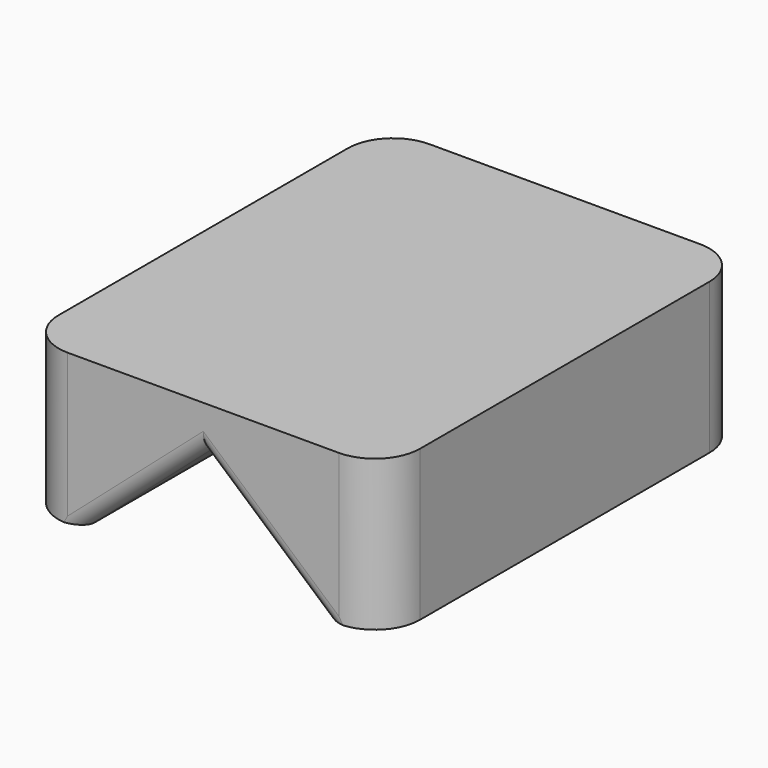
from build123d import *

# Parameters (mm, degrees)
F1_DEPTH     = 15
F2_R         = 1.5
F3_T4_DEPTH  = 7.8150729064
F3_T9_DEPTH  = 7.8150729064
F3_T14_DEPTH = 7.8150729064
F3_T19_DEPTH = 7.8150729064
F3_T25_DEPTH = 7.8150729064
F3_T29_DEPTH = 7.8150729064
F3_T36_DEPTH = 7.8150729064
F3_T40_DEPTH = 7.8150729064


# Not quite as in the source:
# - a fillet or chamfer that OpenCascade refuses, or shapes differently, is made with other operations: its cross-section is extruded or revolved along the edge and cut away or added


with BuildPart() as f1:
    # F0 (on Front) → F1 (new body)
    with BuildSketch(Plane.XZ):
        Polygon((0, 5), (0, 0), (2, 0), (6, 3.5), (10, 0), (12, 0), (12, 5), align=None)
    extrude(amount=F1_DEPTH)

    # F2
    f2_edges = [f1.edges().sort_by_distance(p)[0] for p in [
        (0, -15, 2.5),
        (12, -15, 2.5),
        (12, 0, 2.5),
        (0, 0, 2.5),
    ]]
    fillet(f2_edges, radius=F2_R)

    # F3: fillet of radius 0.5 on 4 edges, made by hand


with BuildPart() as f3_tool2:
    # F3_s3 → F3_t4 (new body)
    with BuildSketch(Plane(origin=(0.1920224944, 0, 0.1680196826), x_dir=(0, 1, 0), z_dir=(0.7525766947, 0, 0.6585046079))):
        with BuildLine():
            ThreePointArc((-15, -0.8170092157), (-14.8535533906, -1.1705626063), (-14.5, -1.3170092157))
            Line((-14.5, -1.3170092157), (-15, -1.3170092157))
            Line((-15, -1.3170092157), (-15, -0.8170092157))
        make_face()
    extrude(amount=F3_T4_DEPTH)

    split(bisect_by=Plane(origin=(4.3362831858, 0, 4.9557522124), x_dir=(0, 1, 0), z_dir=(-0.6585046079, 0, -0.7525766947)), keep=Keep.TOP)


with BuildPart() as f1_1:
    add(f1.part)

    # F3_t1: cut F3_tool2
    add(f3_tool2.part, mode=Mode.SUBTRACT)


with BuildPart() as f3_tool7:
    # F3_s8 → F3_t9 (new body)
    with BuildSketch(Plane(origin=(0.7229959458, 0, -0.6326214526), x_dir=(0, 1, 0), z_dir=(0.7525766947, 0, -0.6585046079))):
        with BuildLine():
            ThreePointArc((-15, 7.0850460787), (-14.8535533906, 6.7314926881), (-14.5, 6.5850460787))
            Line((-14.5, 6.5850460787), (-15, 6.5850460787))
            Line((-15, 6.5850460787), (-15, 7.0850460787))
        make_face()
    extrude(amount=F3_T9_DEPTH)

    split(bisect_by=Plane(origin=(0.8672566372, 0, -0.9911504425), x_dir=(0, 1, 0), z_dir=(0.6585046079, 0, -0.7525766947)), keep=Keep.TOP)


with BuildPart() as f1_2:
    add(f1_1.part)

    # F3_t6: cut F3_tool7
    add(f3_tool7.part, mode=Mode.SUBTRACT)


with BuildPart() as f3_tool12:
    # F3_s13 → F3_t14 (new body)
    with BuildSketch(Plane(origin=(0.1920224944, 0, 0.1680196826), x_dir=(0, 1, 0), z_dir=(0.7525766947, 0, 0.6585046079))):
        with BuildLine():
            ThreePointArc((0, -0.8170092157), (-0.1464466094, -1.1705626063), (-0.5, -1.3170092157))
            Line((-0.5, -1.3170092157), (0, -1.3170092157))
            Line((0, -1.3170092157), (0, -0.8170092157))
        make_face()
    extrude(amount=F3_T14_DEPTH)

    split(bisect_by=Plane(origin=(4.3362831858, 0, 4.9557522124), x_dir=(0, 1, 0), z_dir=(-0.6585046079, 0, -0.7525766947)), keep=Keep.TOP)


with BuildPart() as f1_3:
    add(f1_2.part)

    # F3_t11: cut F3_tool12
    add(f3_tool12.part, mode=Mode.SUBTRACT)


with BuildPart() as f3_tool17:
    # F3_s18 → F3_t19 (new body)
    with BuildSketch(Plane(origin=(0.7229959458, 0, -0.6326214526), x_dir=(0, 1, 0), z_dir=(0.7525766947, 0, -0.6585046079))):
        with BuildLine():
            ThreePointArc((0, 7.0850460787), (-0.1464466094, 6.7314926881), (-0.5, 6.5850460787))
            Line((-0.5, 6.5850460787), (0, 6.5850460787))
            Line((0, 6.5850460787), (0, 7.0850460787))
        make_face()
    extrude(amount=F3_T19_DEPTH)

    split(bisect_by=Plane(origin=(0.8672566372, 0, -0.9911504425), x_dir=(0, 1, 0), z_dir=(0.6585046079, 0, -0.7525766947)), keep=Keep.TOP)


with BuildPart() as f1_4:
    add(f1_3.part)

    # F3_t16: cut F3_tool17
    add(f3_tool17.part, mode=Mode.SUBTRACT)


with BuildPart() as f3_tool23:
    # F3_s24 → F3_t25 (new body)
    with BuildSketch(Plane(origin=(0.1920224944, 0, 0.1680196826), x_dir=(0, 1, 0), z_dir=(0.7525766947, 0, 0.6585046079))):
        with BuildLine():
            ThreePointArc((-15, -0.8170092157), (-14.8535533906, -1.1705626063), (-14.5, -1.3170092157))
            Line((-14.5, -1.3170092157), (-15, -1.3170092157))
            Line((-15, -1.3170092157), (-15, -0.8170092157))
        make_face()
    extrude(amount=F3_T25_DEPTH)

    split(bisect_by=Plane(origin=(4.3362831858, 0, 4.9557522124), x_dir=(0, 1, 0), z_dir=(0.6585046079, 0, 0.7525766947)), keep=Keep.TOP)


with BuildPart() as f3_tool27:
    # F3_s28 → F3_t29 (new body)
    with BuildSketch(Plane(origin=(0.7229959458, 0, -0.6326214526), x_dir=(0, 1, 0), z_dir=(0.7525766947, 0, -0.6585046079))):
        with BuildLine():
            ThreePointArc((-15, 7.0850460787), (-14.8535533906, 6.7314926881), (-14.5, 6.5850460787))
            Line((-14.5, 6.5850460787), (-15, 6.5850460787))
            Line((-15, 6.5850460787), (-15, 7.0850460787))
        make_face()
    extrude(amount=F3_T29_DEPTH)

    split(bisect_by=Plane(origin=(0.8672566372, 0, -0.9911504425), x_dir=(0, 1, 0), z_dir=(-0.6585046079, 0, 0.7525766947)), keep=Keep.TOP)


with BuildPart() as f3_tool23_1:
    add(f3_tool23.part)

    # F3_t31: intersect F3_tool27
    add(f3_tool27.part, mode=Mode.INTERSECT)


with BuildPart() as f1_5:
    add(f1_4.part)

    # F3_t21: cut F3_tool23
    add(f3_tool23_1.part, mode=Mode.SUBTRACT)


with BuildPart() as f3_tool34:
    # F3_s35 → F3_t36 (new body)
    with BuildSketch(Plane(origin=(0.1920224944, 0, 0.1680196826), x_dir=(0, 1, 0), z_dir=(0.7525766947, 0, 0.6585046079))):
        with BuildLine():
            ThreePointArc((0, -0.8170092157), (-0.1464466094, -1.1705626063), (-0.5, -1.3170092157))
            Line((-0.5, -1.3170092157), (0, -1.3170092157))
            Line((0, -1.3170092157), (0, -0.8170092157))
        make_face()
    extrude(amount=F3_T36_DEPTH)

    split(bisect_by=Plane(origin=(4.3362831858, 0, 4.9557522124), x_dir=(0, 1, 0), z_dir=(0.6585046079, 0, 0.7525766947)), keep=Keep.TOP)


with BuildPart() as f3_tool38:
    # F3_s39 → F3_t40 (new body)
    with BuildSketch(Plane(origin=(0.7229959458, 0, -0.6326214526), x_dir=(0, 1, 0), z_dir=(0.7525766947, 0, -0.6585046079))):
        with BuildLine():
            ThreePointArc((0, 7.0850460787), (-0.1464466094, 6.7314926881), (-0.5, 6.5850460787))
            Line((-0.5, 6.5850460787), (0, 6.5850460787))
            Line((0, 6.5850460787), (0, 7.0850460787))
        make_face()
    extrude(amount=F3_T40_DEPTH)

    split(bisect_by=Plane(origin=(0.8672566372, 0, -0.9911504425), x_dir=(0, 1, 0), z_dir=(-0.6585046079, 0, 0.7525766947)), keep=Keep.TOP)


with BuildPart() as f3_tool34_1:
    add(f3_tool34.part)

    # F3_t42: intersect F3_tool38
    add(f3_tool38.part, mode=Mode.INTERSECT)


with BuildPart() as f1_6:
    add(f1_5.part)

    # F3_t32: cut F3_tool34
    add(f3_tool34_1.part, mode=Mode.SUBTRACT)


solid = f1_6.part
